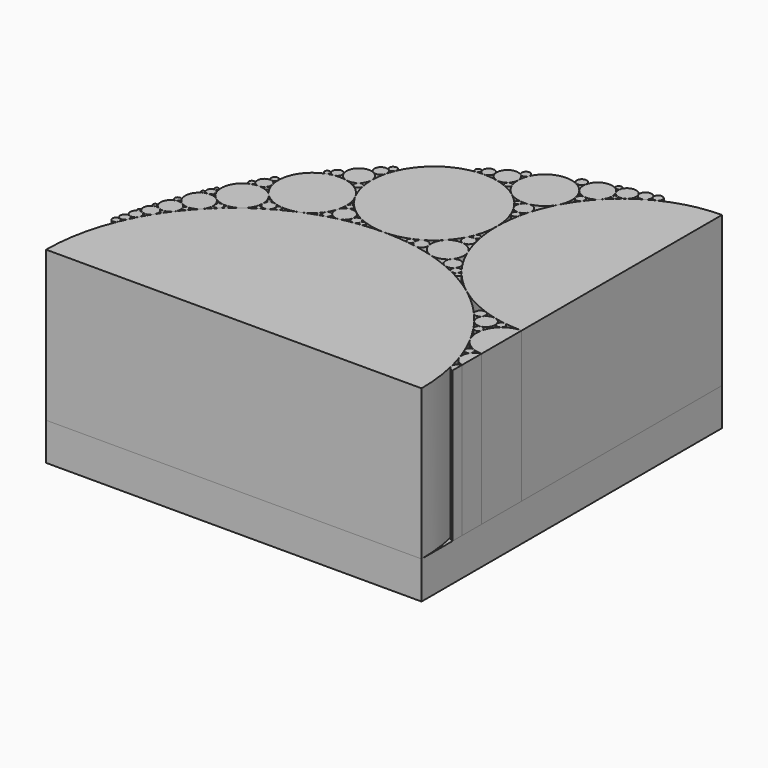
from build123d import *

# Parameters (mm, degrees)
F1_DEPTH = 25
F3_DEPTH = 5


with BuildPart() as f1:
    # F0 (on Top) → F1 (new body)
    with BuildSketch(Plane.XY):
        with BuildLine():
            ThreePointArc((-48.3783783755, 10.2702702693), (-48.7768531909, 10.2270822189), (-49.0099010006, 9.9009900469))
            ThreePointArc((-49.0099010006, 9.9009900469), (-48.6728991311, 9.3351960936), (-48.0769230798, 9.6153846085))
            ThreePointArc((-48.0769230798, 9.6153846085), (-48.0487349636, 9.7077862046), (-48.0392156863, 9.8039215686))
            ThreePointArc((-48.0392156863, 9.8039215686), (-48.1329725068, 10.0922410271), (-48.3783783755, 10.2702702693))
        make_face()
        with BuildLine():
            ThreePointArc((-48.7804878229, 10.9756096761), (-48.7161098211, 10.5450214549), (-48.3783783755, 10.2702702693))
            ThreePointArc((-48.3783783755, 10.2702702693), (-47.952574584, 10.2909216736), (-47.6470587808, 10.5882353855))
            ThreePointArc((-47.6470587808, 10.5882353855), (-47.6047065793, 10.7126925445), (-47.5903614458, 10.843373494))
            ThreePointArc((-47.5903614458, 10.843373494), (-47.6992577773, 11.188832592), (-47.9865768473, 11.4093958515))
            ThreePointArc((-47.9865768473, 11.4093958515), (-48.4816178712, 11.3720178984), (-48.7804878229, 10.9756096761))
        make_face()
        with BuildLine():
            ThreePointArc((-48.4615384416, 12.3076923861), (-48.3969961179, 11.7671053456), (-47.9865768473, 11.4093958515))
            ThreePointArc((-47.9865768473, 11.4093958515), (-47.4563276725, 11.4137449448), (-47.0588235396, 11.7647058633))
            ThreePointArc((-47.0588235396, 11.7647058633), (-46.9923162904, 11.9374730009), (-46.9696969697, 12.1212121212))
            ThreePointArc((-46.9696969697, 12.1212121212), (-46.9898354781, 12.294726766), (-47.0491803261, 12.4590163898))
            ThreePointArc((-47.0491803261, 12.4590163898), (-47.2099365327, 12.6746416924), (-47.4358976334, 12.8205129028))
            ThreePointArc((-47.4358976334, 12.8205129028), (-47.7028475017, 12.8783940259), (-47.9729727653, 12.837837909))
            ThreePointArc((-47.9729727653, 12.837837909), (-48.2843605012, 12.6346069407), (-48.4615384416, 12.3076923861))
        make_face()
        with BuildLine():
            ThreePointArc((-48.253275112, 13.1004366709), (-48.1921054719, 12.8848310695), (-47.9729727653, 12.837837909))
            ThreePointArc((-47.9729727653, 12.837837909), (-47.8665796164, 12.9171222211), (-47.8260869565, 13.0434782609))
            ThreePointArc((-47.8260869565, 13.0434782609), (-47.8359825904, 13.1083205768), (-47.8647685951, 13.1672596592))
            ThreePointArc((-47.8647685951, 13.1672596592), (-48.0803283791, 13.2577235595), (-48.253275112, 13.1004366709))
        make_face()
        with BuildLine():
            ThreePointArc((-47.0491803261, 12.4590163898), (-46.8680978206, 12.3431873313), (-46.6804979568, 12.4481327252))
            ThreePointArc((-46.6804979568, 12.4481327252), (-46.6597834936, 12.4983969045), (-46.6527196653, 12.5523012552))
            ThreePointArc((-46.6527196653, 12.5523012552), (-46.7267903253, 12.7120054984), (-46.8965517221, 12.75862069))
            ThreePointArc((-46.8965517221, 12.75862069), (-47.0483346232, 12.6472648069), (-47.0491803261, 12.4590163898))
        make_face()
        with BuildLine():
            ThreePointArc((-15.3740825035, 23.0725315549), (-16.6741166714, 23.5728586896), (-17.999999924, 23.9999999778))
            ThreePointArc((-17.999999924, 23.9999999778), (-19.2383403471, 24.327007174), (-20.4918032434, 24.590163928))
            ThreePointArc((-20.4918032434, 24.590163928), (-21.0854736332, 24.6916277982), (-21.6814159479, 24.7787610645))
            ThreePointArc((-21.6814159479, 24.7787610645), (-23.337024747, 24.9446289471), (-25.0000000013, 25))
            ThreePointArc((-25.0000000013, 25), (-26.4680505479, 24.9568593294), (-27.9310344796, 24.8275862073))
            ThreePointArc((-27.9310344796, 24.8275862073), (-28.3778301431, 24.7707541977), (-28.8235294642, 24.7058823448))
            ThreePointArc((-28.8235294642, 24.7058823448), (-29.6583413493, 24.5621630944), (-30.4878049658, 24.3902438827))
            ThreePointArc((-30.4878049658, 24.3902438827), (-31.2469504926, 24.2069330883), (-31.9999999474, 24.0000000153))
            ThreePointArc((-31.9999999474, 24.0000000153), (-32.3521462014, 23.8944752241), (-32.7027027159, 23.7837837795))
            ThreePointArc((-32.7027027159, 23.7837837795), (-33.6662535698, 23.449862453), (-34.6153846971, 23.0769230429))
            ThreePointArc((-34.6153846971, 23.0769230429), (-35.7021586706, 22.5934459476), (-36.7647059061, 22.0588235167))
            ThreePointArc((-36.7647059061, 22.0588235167), (-37.2312743797, 21.8035760152), (-37.6923077137, 21.5384615259))
            ThreePointArc((-37.6923077137, 21.5384615259), (-38.1162405871, 21.2829563938), (-38.5350318532, 21.0191082764))
            ThreePointArc((-38.5350318532, 21.0191082764), (-39.2766122189, 20.5226300349), (-40.0000000215, 19.9999999839))
            ThreePointArc((-40.0000000215, 19.9999999839), (-40.6173762093, 19.5217202198), (-41.2195122144, 19.0243902275))
            ThreePointArc((-41.2195122144, 19.0243902275), (-41.4877031588, 18.7924358333), (-41.7525773254, 18.5567010257))
            ThreePointArc((-41.7525773254, 18.5567010257), (-41.9984890871, 18.331703924), (-42.2413792983, 18.1034482874))
            ThreePointArc((-42.2413792983, 18.1034482874), (-42.6776695726, 17.6776694868), (-43.103448371, 17.2413792104))
            ThreePointArc((-43.103448371, 17.2413792104), (-43.6414025747, 16.6582745219), (-44.1605839673, 16.0583941299))
            ThreePointArc((-44.1605839673, 16.0583941299), (-44.5874419484, 15.5348678114), (-44.9999999204, 15.0000001062))
            ThreePointArc((-44.9999999204, 15.0000001062), (-45.3433367345, 14.5309549069), (-45.6756756619, 14.0540540743))
            ThreePointArc((-45.6756756619, 14.0540540743), (-45.9553201945, 13.6335819045), (-46.2264150264, 13.2075472789))
            ThreePointArc((-46.2264150264, 13.2075472789), (-46.4568164706, 12.8298490617), (-46.6804979568, 12.4481327252))
            ThreePointArc((-46.6804979568, 12.4481327252), (-46.8723302213, 12.1078970383), (-47.0588235396, 11.7647058633))
            ThreePointArc((-47.0588235396, 11.7647058633), (-47.3606797573, 11.180339923), (-47.6470587808, 10.5882353855))
            ThreePointArc((-47.6470587808, 10.5882353855), (-47.8671650835, 10.1040962508), (-48.0769230798, 9.6153846085))
            ThreePointArc((-48.0769230798, 9.6153846085), (-49.514516893, 4.9029033748), (-50, 0))
            Line((-50, 0), (0, 0))
            ThreePointArc((0, 0), (-0.1691062282, 2.902880379), (-0.6741371596, 5.7664891458))
            ThreePointArc((-0.6741371596, 5.7664891458), (-0.9478330339, 6.8185969402), (-1.2670102183, 7.857811147))
            ThreePointArc((-1.2670102183, 7.857811147), (-1.5625850115, 8.6998608413), (-1.8880251519, 9.5308246558))
            ThreePointArc((-1.8880251519, 9.5308246558), (-2.3869990459, 10.6607780133), (-2.9411765047, 11.7647059462))
            ThreePointArc((-2.9411765047, 11.7647059462), (-3.5554744724, 12.850382286), (-4.2231626217, 13.904065181))
            ThreePointArc((-4.2231626217, 13.904065181), (-4.6710139033, 14.5510248533), (-5.1390031627, 15.1835702201))
            ThreePointArc((-5.1390031627, 15.1835702201), (-5.6818380323, 15.868478761), (-6.2482802956, 16.5339955282))
            ThreePointArc((-6.2482802956, 16.5339955282), (-8.0353915667, 18.3630623999), (-10.0000002057, 20.0000001543))
            ThreePointArc((-10.0000002057, 20.0000001543), (-11.574433504, 21.089195439), (-13.2275983322, 22.0547173859))
            ThreePointArc((-13.2275983322, 22.0547173859), (-13.6284242829, 22.2640352522), (-14.0329705658, 22.466069202))
            ThreePointArc((-14.0329705658, 22.466069202), (-14.6990624228, 22.7791721762), (-15.3740825035, 23.0725315549))
        make_face()
        with BuildLine():
            ThreePointArc((-47.8647685951, 13.1672596592), (-47.6752178165, 12.9631078353), (-47.4358976334, 12.8205129028))
            ThreePointArc((-47.4358976334, 12.8205129028), (-47.1705941345, 12.751490138), (-46.8965517221, 12.75862069))
            ThreePointArc((-46.8965517221, 12.75862069), (-46.513176207, 12.9109732958), (-46.2264150264, 13.2075472789))
            ThreePointArc((-46.2264150264, 13.2075472789), (-46.1161529749, 13.4561558188), (-46.0784313725, 13.7254901961))
            ThreePointArc((-46.0784313725, 13.7254901961), (-46.0974699197, 13.9177608864), (-46.15384613, 14.1025640453))
            ThreePointArc((-46.15384613, 14.1025640453), (-46.345500421, 14.3980516611), (-46.6292131166, 14.6067413943))
            ThreePointArc((-46.6292131166, 14.6067413943), (-46.975686167, 14.7023509642), (-47.3333331973, 14.6666667064))
            ThreePointArc((-47.3333331973, 14.6666667064), (-47.7520654308, 14.4187321794), (-48.0000000073, 13.9999999751))
            ThreePointArc((-48.0000000073, 13.9999999751), (-48.0265386375, 13.5683397878), (-47.8647685951, 13.1672596592))
        make_face()
        with BuildLine():
            ThreePointArc((-47.6878612564, 15.0289017827), (-47.6191576596, 14.7415335746), (-47.3333331973, 14.6666667064))
            ThreePointArc((-47.3333331973, 14.6666667064), (-47.1839080035, 14.7701149992), (-47.1264367816, 14.9425287356))
            ThreePointArc((-47.1264367816, 14.9425287356), (-47.1374931016, 15.0214715294), (-47.1698112559, 15.0943395183))
            ThreePointArc((-47.1698112559, 15.0943395183), (-47.449804501, 15.2276196596), (-47.6878612564, 15.0289017827))
        make_face()
        with BuildLine():
            ThreePointArc((-45.6284153005, 14.2076502732), (-45.7178489827, 14.4098197098), (-45.927601862, 14.4796380041))
            ThreePointArc((-45.927601862, 14.4796380041), (-46.1359270583, 14.348222835), (-46.15384613, 14.1025640453))
            ThreePointArc((-46.15384613, 14.1025640453), (-45.9292161359, 13.9358214693), (-45.6756756619, 14.0540540743))
            ThreePointArc((-45.6756756619, 14.0540540743), (-45.640497535, 14.1272989601), (-45.6284153005, 14.2076502732))
        make_face()
        with BuildLine():
            ThreePointArc((-44.7976878293, 16.1849709968), (-45.0227558389, 16.6084107386), (-45.3846150972, 16.9230767537))
            ThreePointArc((-45.3846150972, 16.9230767537), (-45.848726574, 17.0893677907), (-46.3414636494, 17.0731706789))
            ThreePointArc((-46.3414636494, 17.0731706789), (-46.9309803896, 16.7691702219), (-47.2972973114, 16.2162161752))
            ThreePointArc((-47.2972973114, 16.2162161752), (-47.3600069048, 15.6409082226), (-47.1698112559, 15.0943395183))
            ThreePointArc((-47.1698112559, 15.0943395183), (-46.9339060797, 14.8124080808), (-46.6292131166, 14.6067413943))
            ThreePointArc((-46.6292131166, 14.6067413943), (-46.2871813171, 14.4947581327), (-45.927601862, 14.4796380041))
            ThreePointArc((-45.927601862, 14.4796380041), (-45.4088802619, 14.6419170708), (-44.9999999204, 15.0000001062))
            ThreePointArc((-44.9999999204, 15.0000001062), (-44.8043640605, 15.3733845814), (-44.7368421053, 15.7894736842))
            ThreePointArc((-44.7368421053, 15.7894736842), (-44.752142495, 15.9895488741), (-44.7976878293, 16.1849709968))
        make_face()
        with BuildLine():
            ThreePointArc((-46.0317460317, 17.4603174603), (-46.0435942475, 17.556561762), (-46.0784313784, 17.6470588345))
            ThreePointArc((-46.0784313784, 17.6470588345), (-46.4543965293, 17.8563016263), (-46.8000000282, 17.599999925))
            ThreePointArc((-46.8000000282, 17.599999925), (-46.7278987508, 17.1997919343), (-46.3414636494, 17.0731706789))
            ThreePointArc((-46.3414636494, 17.0731706789), (-46.1187029285, 17.2124225062), (-46.0317460317, 17.4603174603))
        make_face()
        with BuildLine():
            ThreePointArc((-44.0740740741, 16.2962962963), (-44.1825530447, 16.5581876974), (-44.4444444464, 16.6666666667))
            ThreePointArc((-44.4444444464, 16.6666666667), (-44.7431129935, 16.5153198317), (-44.7976878293, 16.1849709968))
            ThreePointArc((-44.7976878293, 16.1849709968), (-44.5166173118, 15.9330260271), (-44.1605839673, 16.0583941299))
            ThreePointArc((-44.1605839673, 16.0583941299), (-44.096372813, 16.1697247726), (-44.0740740741, 16.2962962963))
        make_face()
        with BuildLine():
            ThreePointArc((-42.7868852266, 19.3442622562), (-43.0218124278, 19.7040451637), (-43.3333333246, 19.9999999935))
            ThreePointArc((-43.3333333246, 19.9999999935), (-43.7149642485, 20.2206389387), (-44.1379310165, 20.3448275832))
            ThreePointArc((-44.1379310165, 20.3448275832), (-44.4137548686, 20.3701160534), (-44.6902652789, 20.3539823287))
            ThreePointArc((-44.6902652789, 20.3539823287), (-44.992254777, 20.2874897226), (-45.2789699655, 20.1716738155))
            ThreePointArc((-45.2789699655, 20.1716738155), (-45.8006217418, 19.7795254255), (-46.1538461805, 19.2307691668))
            ThreePointArc((-46.1538461805, 19.2307691668), (-46.2942002537, 18.4304348801), (-46.0784313784, 17.6470588345))
            ThreePointArc((-46.0784313784, 17.6470588345), (-45.781459528, 17.2372121743), (-45.3846150972, 16.9230767537))
            ThreePointArc((-45.3846150972, 16.9230767537), (-44.9316987396, 16.7319188059), (-44.4444444464, 16.6666666667))
            ThreePointArc((-44.4444444464, 16.6666666667), (-43.7149643262, 16.816398065), (-43.103448371, 17.2413792104))
            ThreePointArc((-43.103448371, 17.2413792104), (-42.7712929298, 17.7248439692), (-42.6070038993, 18.2879376778))
            ThreePointArc((-42.6070038993, 18.2879376778), (-42.5961989308, 18.4030031409), (-42.5925925926, 18.5185185185))
            ThreePointArc((-42.5925925926, 18.5185185185), (-42.6001977638, 18.6861772857), (-42.6229508118, 18.8524589733))
            ThreePointArc((-42.6229508118, 18.8524589733), (-42.6876235083, 19.1041254513), (-42.7868852266, 19.3442622562))
        make_face()
        with BuildLine():
            ThreePointArc((-45.145631068, 20.3883495146), (-45.1610851532, 20.4735736566), (-45.2054794602, 20.5479452148))
            ThreePointArc((-45.2054794602, 20.5479452148), (-45.4240633908, 20.6284260927), (-45.6097560966, 20.4878048801))
            ThreePointArc((-45.6097560966, 20.4878048801), (-45.5560463438, 20.2128786686), (-45.2789699655, 20.1716738155))
            ThreePointArc((-45.2789699655, 20.1716738155), (-45.1816363334, 20.2611413975), (-45.145631068, 20.3883495146))
        make_face()
        with BuildLine():
            ThreePointArc((-44.1860465116, 20.9302325581), (-44.1973367945, 21.0442534571), (-44.2307691446, 21.153845947))
            ThreePointArc((-44.2307691446, 21.153845947), (-44.4242332747, 21.3995175657), (-44.7169811183, 21.5094339611))
            ThreePointArc((-44.7169811183, 21.5094339611), (-45.0579781291, 21.4338288531), (-45.2941176123, 21.1764706626))
            ThreePointArc((-45.2941176123, 21.1764706626), (-45.3431405857, 20.849044324), (-45.2054794602, 20.5479452148))
            ThreePointArc((-45.2054794602, 20.5479452148), (-44.9722846511, 20.3861186153), (-44.6902652789, 20.3539823287))
            ThreePointArc((-44.6902652789, 20.3539823287), (-44.4483275919, 20.4442421927), (-44.2693409849, 20.630372475))
            ThreePointArc((-44.2693409849, 20.630372475), (-44.2072570321, 20.7746256506), (-44.1860465116, 20.9302325581))
        make_face()
        with BuildLine():
            ThreePointArc((-43.9163498099, 20.5323193916), (-43.925003802, 20.58902565), (-43.9501779191, 20.6405693707))
            ThreePointArc((-43.9501779191, 20.6405693707), (-44.1125347083, 20.7223365068), (-44.2693409849, 20.630372475))
            ThreePointArc((-44.2693409849, 20.630372475), (-44.2791670708, 20.4528400463), (-44.1379310165, 20.3448275832))
            ThreePointArc((-44.1379310165, 20.3448275832), (-43.9836611639, 20.387188925), (-43.9163498099, 20.5323193916))
        make_face()
        with BuildLine():
            ThreePointArc((-44.4134078212, 21.7877094972), (-44.4141176802, 21.8076108878), (-44.4162436491, 21.8274111278))
            ThreePointArc((-44.4162436491, 21.8274111278), (-44.6494789119, 22.0636691519), (-44.9438202615, 21.9101122842))
            ThreePointArc((-44.9438202615, 21.9101122842), (-44.9358155097, 21.6500938088), (-44.7169811183, 21.5094339611))
            ThreePointArc((-44.7169811183, 21.5094339611), (-44.5039875289, 21.5818005242), (-44.4134078212, 21.7877094972))
        make_face()
        with BuildLine():
            ThreePointArc((-41.6107382625, 19.127516799), (-41.7754280539, 19.3575112187), (-42.0353982286, 19.4690265485))
            ThreePointArc((-42.0353982286, 19.4690265485), (-42.2847161799, 19.4421460713), (-42.4932975732, 19.3029490769))
            ThreePointArc((-42.4932975732, 19.3029490769), (-42.6110481418, 19.0929357946), (-42.6229508118, 18.8524589733))
            ThreePointArc((-42.6229508118, 18.8524589733), (-42.514954205, 18.6169723615), (-42.3076922708, 18.4615384462))
            ThreePointArc((-42.3076922708, 18.4615384462), (-42.0163348183, 18.4286198686), (-41.7525773254, 18.5567010257))
            ThreePointArc((-41.7525773254, 18.5567010257), (-41.6243097128, 18.7336113301), (-41.5789473684, 18.9473684211))
            ThreePointArc((-41.5789473684, 18.9473684211), (-41.5869560236, 19.038834397), (-41.6107382625, 19.127516799))
        make_face()
        with BuildLine():
            ThreePointArc((-42.4460431655, 19.4244604317), (-42.4795443487, 19.5289996878), (-42.567567597, 19.5945946047))
            ThreePointArc((-42.567567597, 19.5945946047), (-42.7611806376, 19.5429812171), (-42.7868852266, 19.3442622562))
            ThreePointArc((-42.7868852266, 19.3442622562), (-42.6509614223, 19.2463590246), (-42.4932975732, 19.3029490769))
            ThreePointArc((-42.4932975732, 19.3029490769), (-42.4582725373, 19.3592722648), (-42.4460431655, 19.4244604317))
        make_face()
        with BuildLine():
            ThreePointArc((-38.9999999944, 22.9999999808), (-39.2593820819, 23.6082345997), (-39.6551724764, 24.1379311002))
            ThreePointArc((-39.6551724764, 24.1379311002), (-40.187635827, 24.5735021201), (-40.8108108272, 24.8648648702))
            ThreePointArc((-40.8108108272, 24.8648648702), (-41.2334373044, 24.9660082384), (-41.6666666667, 25))
            ThreePointArc((-41.6666666667, 25), (-42.1494037022, 24.9577321084), (-42.6174496585, 24.8322147673))
            ThreePointArc((-42.6174496585, 24.8322147673), (-43.4880184529, 24.3195364699), (-44.1176470189, 23.5294118396))
            ThreePointArc((-44.1176470189, 23.5294118396), (-44.4026583979, 22.7022207943), (-44.4162436491, 21.8274111278))
            ThreePointArc((-44.4162436491, 21.8274111278), (-44.3447667143, 21.484774246), (-44.2307691446, 21.153845947))
            ThreePointArc((-44.2307691446, 21.153845947), (-44.1040223917, 20.8898009479), (-43.9501779191, 20.6405693707))
            ThreePointArc((-43.9501779191, 20.6405693707), (-43.6675561346, 20.2954397436), (-43.3333333246, 19.9999999935))
            ThreePointArc((-43.3333333246, 19.9999999935), (-42.9663547878, 19.7672557926), (-42.567567597, 19.5945946047))
            ThreePointArc((-42.567567597, 19.5945946047), (-42.3045800624, 19.5186845616), (-42.0353982286, 19.4690265485))
            ThreePointArc((-42.0353982286, 19.4690265485), (-41.719399778, 19.4449450301), (-41.4027149338, 19.4570135745))
            ThreePointArc((-41.4027149338, 19.4570135745), (-40.663905284, 19.6317552774), (-40.0000000215, 19.9999999839))
            ThreePointArc((-40.0000000215, 19.9999999839), (-39.3999320164, 20.6166184704), (-39.0173410526, 21.3872831985))
            ThreePointArc((-39.0173410526, 21.3872831985), (-38.9211897318, 21.7998411349), (-38.8888888889, 22.2222222222))
            ThreePointArc((-38.8888888889, 22.2222222222), (-38.9168069606, 22.615059313), (-38.9999999944, 22.9999999808))
        make_face()
        with BuildLine():
            ThreePointArc((-41.1330049261, 19.2118226601), (-41.2136273913, 19.3940739103), (-41.4027149338, 19.4570135745))
            ThreePointArc((-41.4027149338, 19.4570135745), (-41.5875816412, 19.3433119236), (-41.6107382625, 19.127516799))
            ThreePointArc((-41.6107382625, 19.127516799), (-41.4420915446, 18.9736528042), (-41.2195122144, 19.0243902275))
            ThreePointArc((-41.2195122144, 19.0243902275), (-41.1556750338, 19.1086063487), (-41.1330049261, 19.2118226601))
        make_face()
        with BuildLine():
            ThreePointArc((-42.1739130435, 18.2608695652), (-42.210423838, 18.3814565478), (-42.3076922708, 18.4615384462))
            ThreePointArc((-42.3076922708, 18.4615384462), (-42.500373509, 18.4489198173), (-42.6070038993, 18.2879376778))
            ThreePointArc((-42.6070038993, 18.2879376778), (-42.4892362378, 18.0667862735), (-42.2413792983, 18.1034482874))
            ThreePointArc((-42.2413792983, 18.1034482874), (-42.1914902076, 18.1752349428), (-42.1739130435, 18.2608695652))
        make_face()
        with BuildLine():
            ThreePointArc((-38.3870967742, 21.2903225806), (-38.4256544848, 21.4432580092), (-38.532110095, 21.5596330297))
            ThreePointArc((-38.532110095, 21.5596330297), (-38.8176467598, 21.5942977345), (-39.0173410526, 21.3872831985))
            ThreePointArc((-39.0173410526, 21.3872831985), (-38.9054110262, 21.0339115283), (-38.5350318532, 21.0191082764))
            ThreePointArc((-38.5350318532, 21.0191082764), (-38.4264853008, 21.1358541483), (-38.3870967742, 21.2903225806))
        make_face()
        with BuildLine():
            ThreePointArc((-37.3096446599, 22.33502531), (-37.4839253519, 22.7283628273), (-37.8378378275, 22.9729729694))
            ThreePointArc((-37.8378378275, 22.9729729694), (-38.2190179162, 23.0061610835), (-38.5714285813, 22.8571428497))
            ThreePointArc((-38.5714285813, 22.8571428497), (-38.805100948, 22.5771536417), (-38.8888888889, 22.2222222222))
            ThreePointArc((-38.8888888889, 22.2222222222), (-38.7940246834, 21.8459525231), (-38.532110095, 21.5596330297))
            ThreePointArc((-38.532110095, 21.5596330297), (-38.1152397578, 21.4288235105), (-37.6923077137, 21.5384615259))
            ThreePointArc((-37.6923077137, 21.5384615259), (-37.4061562426, 21.8284611493), (-37.3015873016, 22.2222222222))
            ThreePointArc((-37.3015873016, 22.2222222222), (-37.3036042039, 22.2787674644), (-37.3096446599, 22.33502531))
        make_face()
        with BuildLine():
            ThreePointArc((-38.4615384615, 23.0769230769), (-38.4989618306, 23.215349166), (-38.6010362354, 23.316062157))
            ThreePointArc((-38.6010362354, 23.316062157), (-38.9068581382, 23.2922635668), (-38.9999999944, 22.9999999808))
            ThreePointArc((-38.9999999944, 22.9999999808), (-38.8231394925, 22.816295796), (-38.5714285813, 22.8571428497))
            ThreePointArc((-38.5714285813, 22.8571428497), (-38.4905419833, 22.9540621935), (-38.4615384615, 23.0769230769))
        make_face()
        with BuildLine():
            ThreePointArc((-36.5671641791, 22.3880597015), (-36.6614144461, 22.6359566706), (-36.8965517622, 22.7586206942))
            ThreePointArc((-36.8965517622, 22.7586206942), (-37.2074351876, 22.6485730815), (-37.3096446599, 22.33502531))
            ThreePointArc((-37.3096446599, 22.33502531), (-37.1089904376, 22.0552350334), (-36.7647059061, 22.0588235167))
            ThreePointArc((-36.7647059061, 22.0588235167), (-36.6203384675, 22.1960836618), (-36.5671641791, 22.3880597015))
        make_face()
        with BuildLine():
            ThreePointArc((-40.4191616766, 25.1497005988), (-40.4268289796, 25.2170237884), (-40.4494381879, 25.2808988469))
            ThreePointArc((-40.4494381879, 25.2808988469), (-40.6838432464, 25.4470818769), (-40.9502262824, 25.3393664693))
            ThreePointArc((-40.9502262824, 25.3393664693), (-41.0058216154, 25.0652998123), (-40.8108108272, 24.8648648702))
            ThreePointArc((-40.8108108272, 24.8648648702), (-40.5424635705, 24.9075640415), (-40.4191616766, 25.1497005988))
        make_face()
        with BuildLine():
            ThreePointArc((-42.3664122137, 25.1908396947), (-42.3832904577, 25.3030862115), (-42.4324324438, 25.4054054222))
            ThreePointArc((-42.4324324438, 25.4054054222), (-42.7603973831, 25.5723206562), (-43.0769230084, 25.384615501))
            ThreePointArc((-43.0769230084, 25.384615501), (-43.0415305375, 24.946764403), (-42.6174496585, 24.8322147673))
            ThreePointArc((-42.6174496585, 24.8322147673), (-42.4354076621, 24.9719609398), (-42.3664122137, 25.1908396947))
        make_face()
        with BuildLine():
            ThreePointArc((-40.7407407407, 25.9259259259), (-40.7478908475, 26.0407728432), (-40.7692307399, 26.1538460382))
            ThreePointArc((-40.7692307399, 26.1538460382), (-41.0209677006, 26.5895611161), (-41.4634149434, 26.8292683623))
            ThreePointArc((-41.4634149434, 26.8292683623), (-42.0242020677, 26.7800378959), (-42.452830175, 26.4150943616))
            ThreePointArc((-42.452830175, 26.4150943616), (-42.5924037057, 25.9072241907), (-42.4324324438, 25.4054054222))
            ThreePointArc((-42.4324324438, 25.4054054222), (-42.0998960464, 25.1076037859), (-41.6666666667, 25))
            ThreePointArc((-41.6666666667, 25), (-41.2702904487, 25.0891316178), (-40.9502262824, 25.3393664693))
            ThreePointArc((-40.9502262824, 25.3393664693), (-40.7946834253, 25.6145033078), (-40.7407407407, 25.9259259259))
        make_face()
        with BuildLine():
            ThreePointArc((-41.4634149434, 26.8292683623), (-41.079684193, 26.9177868058), (-40.9090909091, 27.2727272727))
            ThreePointArc((-40.9090909091, 27.2727272727), (-41.2330236571, 27.7081028475), (-41.7431192301, 27.5229358343))
            ThreePointArc((-41.7431192301, 27.5229358343), (-41.7852007406, 27.1027418429), (-41.4634149434, 26.8292683623))
        make_face()
        with BuildLine():
            ThreePointArc((-32.5688073907, 24.7706421242), (-32.2383522275, 25.3640136166), (-32.0000000251, 25.9999999141))
            ThreePointArc((-32.0000000251, 25.9999999141), (-31.8638659442, 26.6299028819), (-31.8181818182, 27.2727272727))
            ThreePointArc((-31.8181818182, 27.2727272727), (-31.8282492829, 27.5750864176), (-31.8584070813, 27.8761062068))
            ThreePointArc((-31.8584070813, 27.8761062068), (-32.0369974405, 28.6660515901), (-32.3529410976, 29.411764558))
            ThreePointArc((-32.3529410976, 29.411764558), (-33.0442207872, 30.3779868843), (-33.9622641429, 31.1320754667))
            ThreePointArc((-33.9622641429, 31.1320754667), (-34.6398935726, 31.4786597276), (-35.365853701, 31.7073170827))
            ThreePointArc((-35.365853701, 31.7073170827), (-36.2096416995, 31.81557249), (-37.0588236621, 31.7647058618))
            ThreePointArc((-37.0588236621, 31.7647058618), (-37.4945586834, 31.6752460667), (-37.9194630716, 31.5436241668))
            ThreePointArc((-37.9194630716, 31.5436241668), (-39.0720314963, 30.9231728387), (-40.000000044, 29.9999999413))
            ThreePointArc((-40.000000044, 29.9999999413), (-40.6758331846, 28.7101261744), (-40.9090909091, 27.2727272727))
            ThreePointArc((-40.9090909091, 27.2727272727), (-40.8739903413, 26.7089329654), (-40.7692307399, 26.1538460382))
            ThreePointArc((-40.7692307399, 26.1538460382), (-40.6317110535, 25.7091750776), (-40.4494381879, 25.2808988469))
            ThreePointArc((-40.4494381879, 25.2808988469), (-40.0963126926, 24.6788335879), (-39.6551724764, 24.1379311002))
            ThreePointArc((-39.6551724764, 24.1379311002), (-39.1584799049, 23.6880366857), (-38.6010362354, 23.316062157))
            ThreePointArc((-38.6010362354, 23.316062157), (-38.2273486983, 23.1269181408), (-37.8378378275, 22.9729729694))
            ThreePointArc((-37.8378378275, 22.9729729694), (-37.3729015663, 22.8407366618), (-36.8965517622, 22.7586206942))
            ThreePointArc((-36.8965517622, 22.7586206942), (-35.7354726451, 22.7708868305), (-34.6153846971, 23.0769230429))
            ThreePointArc((-34.6153846971, 23.0769230429), (-33.7387967187, 23.5617470972), (-32.989690653, 24.2268041998))
            ThreePointArc((-32.989690653, 24.2268041998), (-32.7689496543, 24.4907523471), (-32.5688073907, 24.7706421242))
        make_face()
        with BuildLine():
            ThreePointArc((-32.989690653, 24.2268041998), (-33.0161986121, 23.8951670061), (-32.7027027159, 23.7837837795))
            ThreePointArc((-32.7027027159, 23.7837837795), (-32.5659191067, 23.8830131918), (-32.5136612022, 24.043715847))
            ThreePointArc((-32.5136612022, 24.043715847), (-32.5260983853, 24.1252118065), (-32.5622776513, 24.1992883591))
            ThreePointArc((-32.5622776513, 24.1992883591), (-32.7693320633, 24.3163754587), (-32.989690653, 24.2268041998))
        make_face()
        with BuildLine():
            ThreePointArc((-31.6326530612, 24.4897959184), (-31.6633707161, 24.6641546619), (-31.7518248692, 24.8175183099))
            ThreePointArc((-31.7518248692, 24.8175183099), (-32.172083166, 24.999162235), (-32.5688073907, 24.7706421242))
            ThreePointArc((-32.5688073907, 24.7706421242), (-32.6530279085, 24.4839654114), (-32.5622776513, 24.1992883591))
            ThreePointArc((-32.5622776513, 24.1992883591), (-32.3133000292, 24.0089035942), (-31.9999999474, 24.0000000153))
            ThreePointArc((-31.9999999474, 24.0000000153), (-31.7346938611, 24.1836734913), (-31.6326530612, 24.4897959184))
        make_face()
        with BuildLine():
            ThreePointArc((-29.4871794872, 25.641025641), (-29.6225292462, 26.2143764123), (-30.0000000141, 26.6666666772))
            ThreePointArc((-30.0000000141, 26.6666666772), (-30.5813478927, 26.9092352115), (-31.2080537171, 26.8456375745))
            ThreePointArc((-31.2080537171, 26.8456375745), (-31.7049979918, 26.5173789915), (-32.0000000251, 25.9999999141))
            ThreePointArc((-32.0000000251, 25.9999999141), (-32.0239458852, 25.3776903652), (-31.7518248692, 24.8175183099))
            ThreePointArc((-31.7518248692, 24.8175183099), (-31.1797793097, 24.426486475), (-30.4878049658, 24.3902438827))
            ThreePointArc((-30.4878049658, 24.3902438827), (-29.8447375716, 24.7527870371), (-29.5081967159, 25.4098360951))
            ThreePointArc((-29.5081967159, 25.4098360951), (-29.4924446057, 25.5249541867), (-29.4871794872, 25.641025641))
        make_face()
        with BuildLine():
            ThreePointArc((-28.313253012, 25.3012048193), (-28.4048202982, 25.6204812883), (-28.6516853913, 25.8426966283))
            ThreePointArc((-28.6516853913, 25.8426966283), (-29.1873784101, 25.8388551877), (-29.5081967159, 25.4098360951))
            ThreePointArc((-29.5081967159, 25.4098360951), (-29.347505192, 24.8811936384), (-28.8235294642, 24.7058823448))
            ThreePointArc((-28.8235294642, 24.7058823448), (-28.4853705725, 24.8796053647), (-28.3185840914, 25.2212387843))
            ThreePointArc((-28.3185840914, 25.2212387843), (-28.3145872595, 25.2611330488), (-28.313253012, 25.3012048193))
        make_face()
        with BuildLine():
            ThreePointArc((-27.6223776224, 25.1748251748), (-27.6855832345, 25.3753364697), (-27.8523489604, 25.5033556927))
            ThreePointArc((-27.8523489604, 25.5033556927), (-28.1530412119, 25.4739732552), (-28.3185840914, 25.2212387843))
            ThreePointArc((-28.3185840914, 25.2212387843), (-28.2211920096, 24.9295240346), (-27.9310344796, 24.8275862073))
            ThreePointArc((-27.9310344796, 24.8275862073), (-27.7106960414, 24.9425301275), (-27.6223776224, 25.1748251748))
        make_face()
        with BuildLine():
            ThreePointArc((-30.9090909091, 27.2727272727), (-30.9416015049, 27.4415412185), (-31.0344827616, 27.5862068996))
            ThreePointArc((-31.0344827616, 27.5862068996), (-31.2699952394, 27.7175226303), (-31.5384615411, 27.6923076912))
            ThreePointArc((-31.5384615411, 27.6923076912), (-31.7418410437, 27.5248637243), (-31.8181818182, 27.2727272727))
            ThreePointArc((-31.8181818182, 27.2727272727), (-31.6243010769, 26.9003491349), (-31.2080537171, 26.8456375745))
            ThreePointArc((-31.2080537171, 26.8456375745), (-30.9912582258, 27.0120625595), (-30.9090909091, 27.2727272727))
        make_face()
        with BuildLine():
            ThreePointArc((-31.3953488372, 27.9069767442), (-31.4088972269, 27.9851945027), (-31.4479637898, 28.054298629))
            ThreePointArc((-31.4479637898, 28.054298629), (-31.7205198015, 28.1202984565), (-31.8584070813, 27.8761062068))
            ThreePointArc((-31.8584070813, 27.8761062068), (-31.7437498811, 27.7053242962), (-31.5384615411, 27.6923076912))
            ThreePointArc((-31.5384615411, 27.6923076912), (-31.4344069091, 27.7779766973), (-31.3953488372, 27.9069767442))
        make_face()
        with BuildLine():
            ThreePointArc((-21.1764705919, 25.2941176705), (-21.4012383063, 25.6180824546), (-21.7948717866, 25.6410256445))
            ThreePointArc((-21.7948717866, 25.6410256445), (-22.0682226575, 25.1664619451), (-21.6814159479, 24.7787610645))
            ThreePointArc((-21.6814159479, 24.7787610645), (-21.3249979315, 24.8862267079), (-21.1711711712, 25.2252252252))
            ThreePointArc((-21.1711711712, 25.2252252252), (-21.1724979804, 25.2597732095), (-21.1764705919, 25.2941176705))
        make_face()
        with BuildLine():
            ThreePointArc((-19.5121951531, 25.609756236), (-20.0023534316, 26.2014594412), (-20.7692307346, 26.1538461742))
            ThreePointArc((-20.7692307346, 26.1538461742), (-21.1048625617, 25.7865138803), (-21.1764705919, 25.2941176705))
            ThreePointArc((-21.1764705919, 25.2941176705), (-20.9464903098, 24.8328655806), (-20.4918032434, 24.590163928))
            ThreePointArc((-20.4918032434, 24.590163928), (-19.7964538848, 24.7726938423), (-19.4915254237, 25.4237288136))
            ThreePointArc((-19.4915254237, 25.4237288136), (-19.4967087073, 25.5173149231), (-19.5121951531, 25.609756236))
        make_face()
        with BuildLine():
            ThreePointArc((-17.0583995456, 28.2352284583), (-18.0916746878, 28.1449602408), (-18.9655171601, 27.5862069819))
            ThreePointArc((-18.9655171601, 27.5862069819), (-19.486545879, 26.6664915481), (-19.5121951531, 25.609756236))
            ThreePointArc((-19.5121951531, 25.609756236), (-18.9757566999, 24.5985316279), (-17.999999924, 23.9999999778))
            ThreePointArc((-17.999999924, 23.9999999778), (-16.7767597319, 24.0017148485), (-15.7480973985, 24.6636614567))
            ThreePointArc((-15.7480973985, 24.6636614567), (-15.3543842536, 25.3274471734), (-15.2173913044, 26.0869565217))
            ThreePointArc((-15.2173913044, 26.0869565217), (-15.2596072335, 26.5132959796), (-15.384615411, 26.9230769864))
            ThreePointArc((-15.384615411, 26.9230769864), (-16.050088449, 27.7978153217), (-17.0583995456, 28.2352284583))
        make_face()
        with BuildLine():
            ThreePointArc((-14.0389021001, 24.3507387415), (-14.1486008573, 24.5245382081), (-14.256148118, 24.6996771776))
            ThreePointArc((-14.256148118, 24.6996771776), (-15.0100875289, 25.0116095083), (-15.7480973985, 24.6636614567))
            ThreePointArc((-15.7480973985, 24.6636614567), (-15.9675533751, 23.7725522169), (-15.3740825035, 23.0725315549))
            ThreePointArc((-15.3740825035, 23.0725315549), (-14.7505882699, 23.0225707069), (-14.2175420393, 23.3498364426))
            ThreePointArc((-14.2175420393, 23.3498364426), (-14.0391776984, 23.6551867121), (-13.9771824007, 24.0033378405))
            ThreePointArc((-13.9771824007, 24.0033378405), (-13.9927321969, 24.1797582952), (-14.0389021001, 24.3507387415))
        make_face()
        with BuildLine():
            ThreePointArc((-13.3254245286, 23.3227969386), (-13.7649841133, 23.5507445848), (-14.2175420393, 23.3498364426))
            ThreePointArc((-14.2175420393, 23.3498364426), (-14.3416552822, 22.8627587071), (-14.0329705658, 22.466069202))
            ThreePointArc((-14.0329705658, 22.466069202), (-13.6601806891, 22.4213513746), (-13.3401112524, 22.6176356889))
            ThreePointArc((-13.3401112524, 22.6176356889), (-13.2441477334, 22.7874156748), (-13.2108677416, 22.9795788417))
            ThreePointArc((-13.2108677416, 22.9795788417), (-13.2402630107, 23.1604945123), (-13.3254245286, 23.3227969386))
        make_face()
        with BuildLine():
            ThreePointArc((-13.3401112524, 22.6176356889), (-13.4169134698, 22.309581523), (-13.2275983322, 22.0547173859))
            ThreePointArc((-13.2275983322, 22.0547173859), (-12.861660982, 22.0638564981), (-12.6812800722, 22.3823787029))
            ThreePointArc((-12.6812800722, 22.3823787029), (-12.7036748952, 22.5093991018), (-12.7681587562, 22.621102018))
            ThreePointArc((-12.7681587562, 22.621102018), (-13.0549496694, 22.7537905309), (-13.3401112524, 22.6176356889))
        make_face()
        with BuildLine():
            ThreePointArc((-16.8505438405, 29.8350344736), (-17.3132334429, 29.7452202234), (-17.6468065113, 29.4122378279))
            ThreePointArc((-17.6468065113, 29.4122378279), (-17.6565483257, 28.671785729), (-17.0583995456, 28.2352284583))
            ThreePointArc((-17.0583995456, 28.2352284583), (-16.4097956628, 28.4199081154), (-16.1279695529, 29.032580635))
            ThreePointArc((-16.1279695529, 29.032580635), (-16.1318879363, 29.1120028699), (-16.1436050289, 29.1906537114))
            ThreePointArc((-16.1436050289, 29.1906537114), (-16.1538822724, 29.2309114503), (-16.1640591244, 29.2711946846))
            ThreePointArc((-16.1640591244, 29.2711946846), (-16.4227186913, 29.6560955934), (-16.8505438405, 29.8350344736))
        make_face()
        with BuildLine():
            ThreePointArc((-16.3935504202, 30.3284568968), (-16.7692616548, 30.671063543), (-17.1997946066, 30.4005462177))
            ThreePointArc((-17.1997946066, 30.4005462177), (-17.1640097469, 30.0320447185), (-16.8505438405, 29.8350344736))
            ThreePointArc((-16.8505438405, 29.8350344736), (-16.52562349, 29.9406229495), (-16.3866679167, 30.2527343224))
            ThreePointArc((-16.3866679167, 30.2527343224), (-16.3883920816, 30.2907516774), (-16.3935504202, 30.3284568968))
        make_face()
        with BuildLine():
            ThreePointArc((-17.1997946066, 30.4005462177), (-16.8010318925, 31.842908422), (-16.6666666667, 33.3333333333))
            ThreePointArc((-16.6666666667, 33.3333333333), (-16.8284943605, 34.9676344156), (-17.3076922733, 36.5384614559))
            ThreePointArc((-17.3076922733, 36.5384614559), (-17.591878709, 37.1496382717), (-17.9245283781, 37.7358491791))
            ThreePointArc((-17.9245283781, 37.7358491791), (-18.2520847156, 38.2231271693), (-18.6131387512, 38.6861314645))
            ThreePointArc((-18.6131387512, 38.6861314645), (-19.2687945322, 39.3829389677), (-19.999999768, 39.999999826))
            ThreePointArc((-19.999999768, 39.999999826), (-20.8655087626, 40.5686928028), (-21.794871883, 41.0256410624))
            ThreePointArc((-21.794871883, 41.0256410624), (-22.4733028795, 41.2743815076), (-23.1707316623, 41.463414624))
            ThreePointArc((-23.1707316623, 41.463414624), (-24.0797372598, 41.6156977864), (-25, 41.6666666667))
            ThreePointArc((-25, 41.6666666667), (-25.504674401, 41.6513708539), (-26.0074961448, 41.6055395664))
            ThreePointArc((-26.0074961448, 41.6055395664), (-28.1091712388, 41.0649242855), (-30.0000011052, 39.9999991711))
            ThreePointArc((-30.0000011052, 39.9999991711), (-31.5779355776, 38.4495045562), (-32.6923077032, 36.5384615124))
            ThreePointArc((-32.6923077032, 36.5384615124), (-32.9056941544, 35.968564705), (-33.0769230761, 35.3846153878))
            ThreePointArc((-33.0769230761, 35.3846153878), (-33.2689823057, 34.3669561232), (-33.3333333333, 33.3333333333))
            ThreePointArc((-33.3333333333, 33.3333333333), (-33.2919765855, 32.5041356791), (-33.1683168334, 31.6831683253))
            ThreePointArc((-33.1683168334, 31.6831683253), (-32.8432888962, 30.5177936452), (-32.3529410976, 29.411764558))
            ThreePointArc((-32.3529410976, 29.411764558), (-31.9337524015, 28.7108316211), (-31.4479637898, 28.054298629))
            ThreePointArc((-31.4479637898, 28.054298629), (-31.2456100938, 27.8163777417), (-31.0344827616, 27.5862068996))
            ThreePointArc((-31.0344827616, 27.5862068996), (-30.5363653317, 27.1049223516), (-30.0000000141, 26.6666666772))
            ThreePointArc((-30.0000000141, 26.6666666772), (-29.345416752, 26.2226513903), (-28.6516853913, 25.8426966283))
            ThreePointArc((-28.6516853913, 25.8426966283), (-28.2564403541, 25.6626071184), (-27.8523489604, 25.5033556927))
            ThreePointArc((-27.8523489604, 25.5033556927), (-26.4482110993, 25.1268036736), (-25.0000000013, 25))
            ThreePointArc((-25.0000000013, 25), (-23.3656988701, 25.1618277033), (-21.7948717866, 25.6410256445))
            ThreePointArc((-21.7948717866, 25.6410256445), (-21.2732200155, 25.8797734193), (-20.7692307346, 26.1538461742))
            ThreePointArc((-20.7692307346, 26.1538461742), (-19.8176487414, 26.8074096533), (-18.9655171601, 27.5862069819))
            ThreePointArc((-18.9655171601, 27.5862069819), (-18.2441827635, 28.4544627763), (-17.6468065113, 29.4122378279))
            ThreePointArc((-17.6468065113, 29.4122378279), (-17.4072032302, 29.8991112007), (-17.1997946066, 30.4005462177))
        make_face()
        with BuildLine():
            ThreePointArc((-34.0000000446, 31.9999999666), (-33.5092880275, 32.5879773159), (-33.3333333333, 33.3333333333))
            ThreePointArc((-33.3333333333, 33.3333333333), (-33.5866694444, 34.2166648217), (-34.2696627553, 34.8314605932))
            ThreePointArc((-34.2696627553, 34.8314605932), (-35.295254882, 34.973638894), (-36.2068965178, 34.4827586564))
            ThreePointArc((-36.2068965178, 34.4827586564), (-36.6388033159, 33.6368155727), (-36.5384616283, 32.692307908))
            ThreePointArc((-36.5384616283, 32.692307908), (-36.0719869168, 32.0571586478), (-35.365853701, 31.7073170827))
            ThreePointArc((-35.365853701, 31.7073170827), (-34.6507849006, 31.7036626328), (-34.0000000446, 31.9999999666))
        make_face()
        with BuildLine():
            ThreePointArc((-36.4864864865, 32.4324324324), (-36.4996076745, 32.5649434491), (-36.5384616283, 32.692307908))
            ThreePointArc((-36.5384616283, 32.692307908), (-37.0535976368, 33.0993292479), (-37.6712328172, 32.876712397))
            ThreePointArc((-37.6712328172, 32.876712397), (-37.835651316, 32.4867461355), (-37.7358490736, 32.0754717255))
            ThreePointArc((-37.7358490736, 32.0754717255), (-37.4440322786, 31.8183584498), (-37.0588236621, 31.7647058618))
            ThreePointArc((-37.0588236621, 31.7647058618), (-36.6491509881, 31.9927084805), (-36.4864864865, 32.4324324324))
        make_face()
        with BuildLine():
            ThreePointArc((-37.7358490736, 32.0754717255), (-38.0179663196, 32.2454775099), (-38.321167896, 32.1167883059))
            ThreePointArc((-38.321167896, 32.1167883059), (-38.3401822235, 31.6761115817), (-37.9194630716, 31.5436241668))
            ThreePointArc((-37.9194630716, 31.5436241668), (-37.7466550965, 31.6762817661), (-37.6811594203, 31.884057971))
            ThreePointArc((-37.6811594203, 31.884057971), (-37.6951000234, 31.9835946271), (-37.7358490736, 32.0754717255))
        make_face()
        with BuildLine():
            ThreePointArc((-33.1578947368, 31.5789473684), (-33.1605067424, 31.6313177512), (-33.1683168334, 31.6831683253))
            ThreePointArc((-33.1683168334, 31.6831683253), (-33.4968445945, 32.0707830298), (-34.0000000446, 31.9999999666))
            ThreePointArc((-34.0000000446, 31.9999999666), (-34.2100295556, 31.5560856389), (-33.9622641429, 31.1320754667))
            ThreePointArc((-33.9622641429, 31.1320754667), (-33.4286089795, 31.1188645938), (-33.1578947368, 31.5789473684))
        make_face()
        with BuildLine():
            ThreePointArc((-34.2696627553, 34.8314605932), (-33.5417584077, 34.8244167901), (-33.0769230761, 35.3846153878))
            ThreePointArc((-33.0769230761, 35.3846153878), (-33.0573916297, 35.4881061588), (-33.0508474576, 35.593220339))
            ThreePointArc((-33.0508474576, 35.593220339), (-33.1543257792, 35.9990272176), (-33.4394904232, 36.3057324695))
            ThreePointArc((-33.4394904232, 36.3057324695), (-33.9782327, 36.4369003767), (-34.4827586874, 36.2068964882))
            ThreePointArc((-34.4827586874, 36.2068964882), (-34.7357713663, 35.4634719017), (-34.2696627553, 34.8314605932))
        make_face()
        with BuildLine():
            ThreePointArc((-33.4394904232, 36.3057324695), (-33.0115389501, 36.2475724165), (-32.6923077032, 36.5384615124))
            ThreePointArc((-32.6923077032, 36.5384615124), (-32.6629690458, 36.6346346111), (-32.6530612245, 36.7346938776))
            ThreePointArc((-32.6530612245, 36.7346938776), (-32.9560517808, 37.2009242496), (-33.5051546031, 37.1134020944))
            ThreePointArc((-33.5051546031, 37.1134020944), (-33.6717915227, 36.6933502936), (-33.4394904232, 36.3057324695))
        make_face()
        with BuildLine():
            ThreePointArc((-25.69959422, 42.1335725844), (-26.3852976033, 42.1796268254), (-26.0074961448, 41.6055395664))
            ThreePointArc((-26.0074961448, 41.6055395664), (-25.7666681738, 41.7320200503), (-25.670231439, 41.9863729167))
            ThreePointArc((-25.670231439, 41.9863729167), (-25.6776437393, 42.0614227586), (-25.69959422, 42.1335725844))
        make_face()
        with BuildLine():
            ThreePointArc((-25.69959422, 42.1335725844), (-25.4205452439, 41.7941132896), (-25, 41.6666666667))
            ThreePointArc((-25, 41.6666666667), (-24.4643130446, 41.8885554688), (-24.2424242424, 42.4242424242))
            ThreePointArc((-24.2424242424, 42.4242424242), (-24.2461839487, 42.4996240481), (-24.25742575, 42.5742574623))
            ThreePointArc((-24.25742575, 42.5742574623), (-24.6914520089, 43.1161377672), (-25.3846152457, 43.0769231588))
            ThreePointArc((-25.3846152457, 43.0769231588), (-25.7185785398, 42.664171394), (-25.69959422, 42.1335725844))
        make_face()
        with BuildLine():
            ThreePointArc((-24.25742575, 42.5742574623), (-23.8783343192, 41.8581512033), (-23.1707316623, 41.463414624))
            ThreePointArc((-23.1707316623, 41.463414624), (-22.5063205374, 41.4723179489), (-21.9178082399, 41.7808218997))
            ThreePointArc((-21.9178082399, 41.7808218997), (-21.5566193236, 42.2659957813), (-21.4285714286, 42.8571428571))
            ThreePointArc((-21.4285714286, 42.8571428571), (-21.5793897249, 43.4960194177), (-21.999999992, 43.999999994))
            ThreePointArc((-21.999999992, 43.999999994), (-22.7475764318, 44.281506408), (-23.5294117765, 44.1176470525))
            ThreePointArc((-23.5294117765, 44.1176470525), (-24.1491879842, 43.466598119), (-24.25742575, 42.5742574623))
        make_face()
        with BuildLine():
            ThreePointArc((-21.9178082399, 41.7808218997), (-22.0662194964, 41.3690650776), (-21.794871883, 41.0256410624))
            ThreePointArc((-21.794871883, 41.0256410624), (-21.3717567081, 41.0666439851), (-21.1711711712, 41.4414414414))
            ThreePointArc((-21.1711711712, 41.4414414414), (-21.1784369769, 41.5220204645), (-21.1999999978, 41.5999999941))
            ThreePointArc((-21.1999999978, 41.5999999941), (-21.5115869655, 41.8782457257), (-21.9178082399, 41.7808218997))
        make_face()
        with BuildLine():
            ThreePointArc((-21.999999992, 43.999999994), (-21.5204903263, 43.9084645448), (-21.1538461547, 44.2307692288))
            ThreePointArc((-21.1538461547, 44.2307692288), (-21.1218996248, 44.335491035), (-21.1111111111, 44.4444444444))
            ThreePointArc((-21.1111111111, 44.4444444444), (-21.3722228154, 44.915554616), (-21.9101123687, 44.9438202202))
            ThreePointArc((-21.9101123687, 44.9438202202), (-22.219719708, 44.4971161525), (-21.999999992, 43.999999994))
        make_face()
        with BuildLine():
            ThreePointArc((-17.2131146941, 39.3442623061), (-15.7499408109, 39.973603092), (-14.7058824499, 41.1764704064))
            ThreePointArc((-14.7058824499, 41.1764704064), (-14.3923482388, 41.9909440964), (-14.2857142857, 42.8571428571))
            ThreePointArc((-14.2857142857, 42.8571428571), (-14.3034386067, 43.2125132857), (-14.3564356449, 43.5643564424))
            ThreePointArc((-14.3564356449, 43.5643564424), (-14.5981810269, 44.3180568963), (-15.0000001221, 45.0000001628))
            ThreePointArc((-15.0000001221, 45.0000001628), (-15.5825663894, 45.6105777907), (-16.2921349486, 46.0674157874))
            ThreePointArc((-16.2921349486, 46.0674157874), (-17.7521462928, 46.4270276959), (-19.2307692001, 46.1538461666))
            ThreePointArc((-19.2307692001, 46.1538461666), (-20.3825242075, 45.3825242295), (-21.1538461547, 44.2307692288))
            ThreePointArc((-21.1538461547, 44.2307692288), (-21.3592166991, 43.5575576244), (-21.4285714286, 42.8571428571))
            ThreePointArc((-21.4285714286, 42.8571428571), (-21.3709639641, 42.218266289), (-21.1999999978, 41.5999999941))
            ThreePointArc((-21.1999999978, 41.5999999941), (-20.7142856254, 40.7142855957), (-19.999999768, 39.999999826))
            ThreePointArc((-19.999999768, 39.999999826), (-19.183537965, 39.5411546095), (-18.2758620044, 39.31034482))
            ThreePointArc((-18.2758620044, 39.31034482), (-17.7432190356, 39.2875317574), (-17.2131146941, 39.3442623061))
        make_face()
        with BuildLine():
            ThreePointArc((-18.2758620044, 39.31034482), (-18.6564071042, 39.1127361911), (-18.6131387512, 38.6861314645))
            ThreePointArc((-18.6131387512, 38.6861314645), (-18.2741718251, 38.552453958), (-17.9775280887, 38.7640449463))
            ThreePointArc((-17.9775280887, 38.7640449463), (-17.9487056502, 38.8454734721), (-17.9389312977, 38.9312977099))
            ThreePointArc((-17.9389312977, 38.9312977099), (-18.0353399331, 39.1848716699), (-18.2758620044, 39.31034482))
        make_face()
        with BuildLine():
            ThreePointArc((-17.9775280887, 38.7640449463), (-18.0836958829, 38.2431085333), (-17.9245283781, 37.7358491791))
            ThreePointArc((-17.9245283781, 37.7358491791), (-17.4824177326, 37.3391843473), (-16.8965517185, 37.241379311))
            ThreePointArc((-16.8965517185, 37.241379311), (-16.3341040018, 37.4857592681), (-16.000000004, 37.9999999861))
            ThreePointArc((-16.000000004, 37.9999999861), (-15.9681388376, 38.147424082), (-15.9574468085, 38.2978723404))
            ThreePointArc((-15.9574468085, 38.2978723404), (-16.3402293386, 39.1151290013), (-17.2131146941, 39.3442623061))
            ThreePointArc((-17.2131146941, 39.3442623061), (-17.6644643394, 39.1452467221), (-17.9775280887, 38.7640449463))
        make_face()
        with BuildLine():
            ThreePointArc((-16.8965517185, 37.241379311), (-17.2771365534, 36.9922873695), (-17.3076922733, 36.5384614559))
            ThreePointArc((-17.3076922733, 36.5384614559), (-16.7869533269, 36.2269242246), (-16.3366336699, 36.6336633342))
            ThreePointArc((-16.3366336699, 36.6336633342), (-16.3290626597, 36.6839266576), (-16.3265306122, 36.7346938776))
            ThreePointArc((-16.3265306122, 36.7346938776), (-16.4977735495, 37.1160251607), (-16.8965517185, 37.241379311))
        make_face()
        with BuildLine():
            ThreePointArc((-14.3564356449, 43.5643564424), (-13.9196901498, 43.1175626411), (-13.3333333215, 43.3333333491))
            ThreePointArc((-13.3333333215, 43.3333333491), (-13.2478831589, 43.4964208335), (-13.2183908046, 43.6781609195))
            ThreePointArc((-13.2183908046, 43.6781609195), (-13.360588078, 44.0566118111), (-13.7168140736, 44.2477875991))
            ThreePointArc((-13.7168140736, 44.2477875991), (-14.2127130455, 44.0708725296), (-14.3564356449, 43.5643564424))
        make_face()
        with BuildLine():
            ThreePointArc((-13.7168140736, 44.2477875991), (-12.8232572861, 44.3397838635), (-12.0689655779, 44.8275861432))
            ThreePointArc((-12.0689655779, 44.8275861432), (-11.67600638, 45.4396332739), (-11.5384615385, 46.1538461538))
            ThreePointArc((-11.5384615385, 46.1538461538), (-11.5958797944, 46.6202607653), (-11.7647058319, 47.0588234348))
            ThreePointArc((-11.7647058319, 47.0588234348), (-12.0470286007, 47.4566840968), (-12.4203821484, 47.7707006259))
            ThreePointArc((-12.4203821484, 47.7707006259), (-13.185277653, 48.056976422), (-14.0000000897, 47.9999999739))
            ThreePointArc((-14.0000000897, 47.9999999739), (-14.877552994, 47.4550485577), (-15.3465346756, 46.5346533556))
            ThreePointArc((-15.3465346756, 46.5346533556), (-15.3373865525, 45.7302675996), (-15.0000001221, 45.0000001628))
            ThreePointArc((-15.0000001221, 45.0000001628), (-14.4340760115, 44.4948116256), (-13.7168140736, 44.2477875991))
        make_face()
        with BuildLine():
            ThreePointArc((-16.216216151, 47.2972973197), (-16.6654001472, 46.7077408496), (-16.2921349486, 46.0674157874))
            ThreePointArc((-16.2921349486, 46.0674157874), (-15.7046736612, 46.0689821361), (-15.3465346756, 46.5346533556))
            ThreePointArc((-15.3465346756, 46.5346533556), (-15.3366418788, 46.6003307983), (-15.3333333333, 46.6666666667))
            ThreePointArc((-15.3333333333, 46.6666666667), (-15.6125078428, 47.2091556274), (-16.216216151, 47.2972973197))
        make_face()
        with BuildLine():
            ThreePointArc((-12.3076923839, 48.4615384422), (-12.5904410721, 48.1530506211), (-12.4203821484, 47.7707006259))
            ThreePointArc((-12.4203821484, 47.7707006259), (-12.0840482395, 47.7326335775), (-11.8497109771, 47.9768786305))
            ThreePointArc((-11.8497109771, 47.9768786305), (-11.8364993506, 48.0335659694), (-11.8320610687, 48.0916030534))
            ThreePointArc((-11.8320610687, 48.0916030534), (-11.9794120106, 48.3928825499), (-12.3076923839, 48.4615384422))
        make_face()
        with BuildLine():
            ThreePointArc((-11.081081115, 46.4864864975), (-11.394465643, 46.436620998), (-11.5384615385, 46.1538461538))
            ThreePointArc((-11.5384615385, 46.1538461538), (-11.3334975298, 45.8355361953), (-10.9589041044, 45.8904109634))
            ThreePointArc((-10.9589041044, 45.8904109634), (-10.8705012302, 46.0091598128), (-10.8391608392, 46.1538461538))
            ThreePointArc((-10.8391608392, 46.1538461538), (-10.9060363447, 46.359500608), (-11.081081115, 46.4864864975))
        make_face()
        with BuildLine():
            ThreePointArc((-11.8497109771, 47.9768786305), (-11.8996912746, 47.5092878004), (-11.7647058319, 47.0588234348))
            ThreePointArc((-11.7647058319, 47.0588234348), (-11.4784959922, 46.7062408425), (-11.081081115, 46.4864864975))
            ThreePointArc((-11.081081115, 46.4864864975), (-10.5185726567, 46.4447691345), (-10.000000008, 46.6666666606))
            ThreePointArc((-10.000000008, 46.6666666606), (-9.6494914415, 47.0866504771), (-9.5238095238, 47.619047619))
            ThreePointArc((-9.5238095238, 47.619047619), (-9.5469277436, 47.8525190913), (-9.6153845235, 48.0769228563))
            ThreePointArc((-9.6153845235, 48.0769228563), (-10.1673535648, 48.6764495218), (-10.9756097626, 48.7804878034))
            ThreePointArc((-10.9756097626, 48.7804878034), (-11.5199991157, 48.4954376435), (-11.8497109771, 47.9768786305))
        make_face()
        with BuildLine():
            ThreePointArc((-9.6153845235, 48.0769228563), (-9.1259900126, 47.6220295579), (-8.4615384471, 47.6923077008))
            ThreePointArc((-8.4615384471, 47.6923077008), (-8.1707716554, 47.9869847344), (-8.064516129, 48.3870967742))
            ThreePointArc((-8.064516129, 48.3870967742), (-8.075488782, 48.5196766678), (-8.1081081509, 48.6486487735))
            ThreePointArc((-8.1081081509, 48.6486487735), (-8.463565213, 49.083076216), (-9.0163934336, 49.1803278705))
            ThreePointArc((-9.0163934336, 49.1803278705), (-9.5797205642, 48.7718481755), (-9.6153845235, 48.0769228563))
        make_face()
        with BuildLine():
            ThreePointArc((-8.1081081509, 48.6486487735), (-7.7810335922, 48.3002374308), (-7.3033707889, 48.3146067404))
            ThreePointArc((-7.3033707889, 48.3146067404), (-7.0651172658, 48.5290703826), (-6.976744186, 48.8372093023))
            ThreePointArc((-6.976744186, 48.8372093023), (-7.1797724934, 49.2786375904), (-7.6470589174, 49.4117646914))
            ThreePointArc((-7.6470589174, 49.4117646914), (-8.0557648404, 49.137857946), (-8.1081081509, 48.6486487735))
        make_face()
        with BuildLine():
            ThreePointArc((-16.3366336699, 36.6336633342), (-16.5839531718, 34.991728634), (-16.6666666667, 33.3333333333))
            ThreePointArc((-16.6666666667, 33.3333333333), (-16.5982471682, 31.8247019268), (-16.3935504202, 30.3284568968))
            ThreePointArc((-16.3935504202, 30.3284568968), (-16.2873857835, 29.7979631805), (-16.1640591244, 29.2711946846))
            ThreePointArc((-16.1640591244, 29.2711946846), (-16.1527945466, 29.231187688), (-16.1436050289, 29.1906537114))
            ThreePointArc((-16.1436050289, 29.1906537114), (-15.8048298655, 28.0432359145), (-15.384615411, 26.9230769864))
            ThreePointArc((-15.384615411, 26.9230769864), (-14.8620184471, 25.7902447448), (-14.256148118, 24.6996771776))
            ThreePointArc((-14.256148118, 24.6996771776), (-14.1295604447, 24.5363926024), (-14.0389021001, 24.3507387415))
            ThreePointArc((-14.0389021001, 24.3507387415), (-13.6918135777, 23.8300697502), (-13.3254245286, 23.3227969386))
            ThreePointArc((-13.3254245286, 23.3227969386), (-13.0515081926, 22.9682037308), (-12.7681587562, 22.621102018))
            ThreePointArc((-12.7681587562, 22.621102018), (-11.4592674013, 21.2311447542), (-10.0000002057, 20.0000001543))
            ThreePointArc((-10.0000002057, 20.0000001543), (-7.8535504975, 18.6330094471), (-5.5240088006, 17.6087314449))
            ThreePointArc((-5.5240088006, 17.6087314449), (-4.7070151943, 17.3451568977), (-3.877533781, 17.1239993077))
            ThreePointArc((-3.877533781, 17.1239993077), (-3.1300908167, 16.9632292024), (-2.3760613124, 16.8369061317))
            ThreePointArc((-2.3760613124, 16.8369061317), (-1.1910760718, 16.7092810124), (0, 16.6666666667))
            Line((0, 16.6666666667), (0, 50))
            ThreePointArc((0, 50), (-3.7476584463, 49.5731865946), (-7.3033707889, 48.3146067404))
            ThreePointArc((-7.3033707889, 48.3146067404), (-7.8885933365, 48.0148820578), (-8.4615384471, 47.6923077008))
            ThreePointArc((-8.4615384471, 47.6923077008), (-9.2450032676, 47.2008382408), (-10.000000008, 46.6666666606))
            ThreePointArc((-10.000000008, 46.6666666606), (-10.4866371457, 46.2874145108), (-10.9589041044, 45.8904109634))
            ThreePointArc((-10.9589041044, 45.8904109634), (-11.5261916814, 45.3718001419), (-12.0689655779, 44.8275861432))
            ThreePointArc((-12.0689655779, 44.8275861432), (-12.7231047782, 44.0990373317), (-13.3333333215, 43.3333333491))
            ThreePointArc((-13.3333333215, 43.3333333491), (-14.0610248456, 42.2812581246), (-14.7058824499, 41.1764704064))
            ThreePointArc((-14.7058824499, 41.1764704064), (-15.4348727044, 39.6216146865), (-16.000000004, 37.9999999861))
            ThreePointArc((-16.000000004, 37.9999999861), (-16.1827435345, 37.3203860639), (-16.3366336699, 36.6336633342))
        make_face()
        with BuildLine():
            ThreePointArc((-5.5240088006, 17.6087314449), (-6.3013195306, 17.3511525963), (-6.2482802956, 16.5339955282))
            ThreePointArc((-6.2482802956, 16.5339955282), (-5.699791737, 16.3088070002), (-5.1875008388, 16.6073159745))
            ThreePointArc((-5.1875008388, 16.6073159745), (-5.104690686, 16.7839217219), (-5.0762839999, 16.9768988489))
            ThreePointArc((-5.0762839999, 16.9768988489), (-5.1995618926, 17.3640906381), (-5.5240088006, 17.6087314449))
        make_face()
        with BuildLine():
            ThreePointArc((-3.877533781, 17.1239993077), (-4.6139194778, 17.0720396772), (-5.1875008388, 16.6073159745))
            ThreePointArc((-5.1875008388, 16.6073159745), (-5.3907591755, 15.8876934206), (-5.1390031627, 15.1835702201))
            ThreePointArc((-5.1390031627, 15.1835702201), (-4.5822744846, 14.774991253), (-3.8930841612, 14.7313989203))
            ThreePointArc((-3.8930841612, 14.7313989203), (-3.2040283561, 15.1624935678), (-2.9350806795, 15.9295057221))
            ThreePointArc((-2.9350806795, 15.9295057221), (-2.9426188957, 16.0653732218), (-2.9651410108, 16.1995729107))
            ThreePointArc((-2.9651410108, 16.1995729107), (-3.2891398769, 16.7922627604), (-3.877533781, 17.1239993077))
        make_face()
        with BuildLine():
            ThreePointArc((-2.3760613124, 16.8369061317), (-2.8380801044, 16.673038364), (-2.9651410108, 16.1995729107))
            ThreePointArc((-2.9651410108, 16.1995729107), (-2.6221744274, 15.8170840457), (-2.1166219735, 15.9084105229))
            ThreePointArc((-2.1166219735, 15.9084105229), (-1.9748078726, 16.0903443536), (-1.92430979, 16.3154245651))
            ThreePointArc((-1.92430979, 16.3154245651), (-2.0529529457, 16.6603964706), (-2.3760613124, 16.8369061317))
        make_face()
        with BuildLine():
            ThreePointArc((-3.2341022762, 14.2044782943), (-3.4369278912, 14.6263498598), (-3.8930841612, 14.7313989203))
            ThreePointArc((-3.8930841612, 14.7313989203), (-4.2759539045, 14.4046391318), (-4.2231626217, 13.904065181))
            ThreePointArc((-4.2231626217, 13.904065181), (-3.6767760325, 13.6731937), (-3.2479399609, 14.082998006))
            ThreePointArc((-3.2479399609, 14.082998006), (-3.2375728468, 14.1433453614), (-3.2341022762, 14.2044782943))
        make_face()
        with BuildLine():
            Line((0, 10), (0, 16.6666666667))
            ThreePointArc((0, 16.6666666667), (-1.1241709121, 16.471382229), (-2.1166219735, 15.9084105229))
            ThreePointArc((-2.1166219735, 15.9084105229), (-2.8333132374, 15.0893080512), (-3.2479399609, 14.082998006))
            ThreePointArc((-3.2479399609, 14.082998006), (-3.3045287372, 12.8960680404), (-2.9411765047, 11.7647059462))
            ThreePointArc((-2.9411765047, 11.7647059462), (-2.2121042986, 10.8398005617), (-1.2068958591, 10.2261620319))
            ThreePointArc((-1.2068958591, 10.2261620319), (-0.6139517244, 10.0570283428), (0, 10))
        make_face()
        with BuildLine():
            ThreePointArc((-0.8691595474, 9.7326585566), (-0.9616774716, 10.0316616905), (-1.2068958591, 10.2261620319))
            ThreePointArc((-1.2068958591, 10.2261620319), (-1.7767870884, 10.1031340127), (-1.8880251519, 9.5308246558))
            ThreePointArc((-1.8880251519, 9.5308246558), (-1.4746095339, 9.2087215744), (-0.9866943206, 9.4000370542))
            ThreePointArc((-0.9866943206, 9.4000370542), (-0.8994073189, 9.5562701452), (-0.8691595474, 9.7326585566))
        make_face()
        with BuildLine():
            Line((0, 6.7611418346), (0, 9.9830179351))
            ThreePointArc((0, 9.9830179351), (-0.5460598119, 9.7807435834), (-0.9866943206, 9.4000370542))
            ThreePointArc((-0.9866943206, 9.4000370542), (-1.3235567402, 8.6646772221), (-1.2670102183, 7.857811147))
            ThreePointArc((-1.2670102183, 7.857811147), (-0.7845552271, 7.1349644107), (0, 6.7611418346))
        make_face()
        with BuildLine():
            Line((0, 5.1619892342), (0, 6.7371152955))
            ThreePointArc((0, 6.7371152955), (-0.5537397606, 6.4022886818), (-0.6741371596, 5.7664891458))
            ThreePointArc((-0.6741371596, 5.7664891458), (-0.4317342848, 5.3586681746), (0, 5.1619892342))
        make_face()
    extrude(amount=F1_DEPTH)


with BuildPart() as f3:
    # F2 (on Top) → F3 (new body)
    with BuildSketch(Plane.XY):
        with BuildLine():
            Line((-50, 0), (0, 0))
            Line((0, 0), (0, 50))
            ThreePointArc((0, 50), (-35.3553390593, 35.3553390593), (-50, 0))
        make_face()
    extrude(amount=F3_DEPTH)


solid = Compound([f1.part, f3.part])
